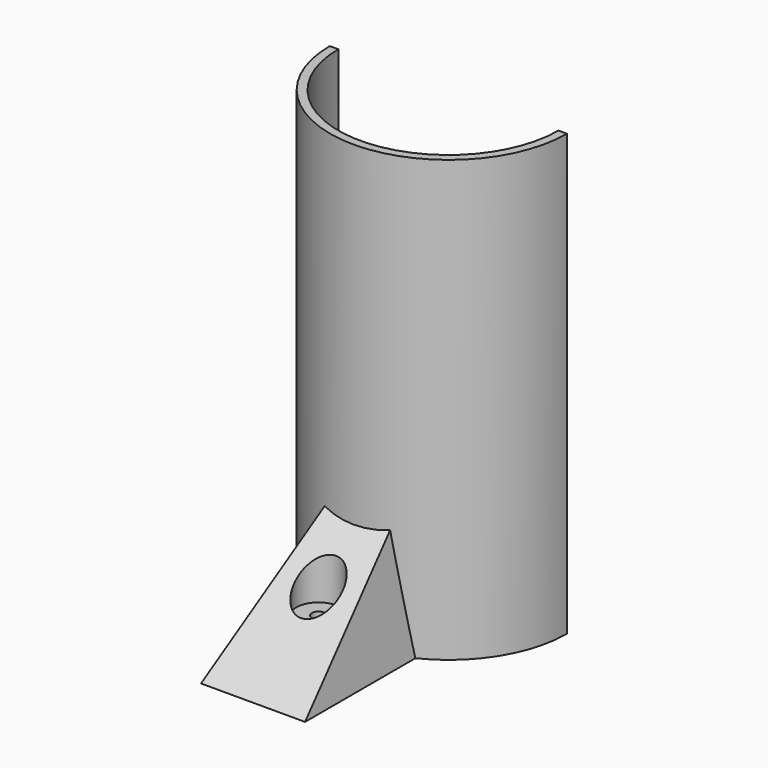
from build123d import *

# Parameters (mm, degrees)
F1_DEPTH               = 50
F2_DEPTH               = 50
DRAFT_F2_DRAFTED_ANGLE = -10
F3_T4_DEPTH            = 268.8954225412
F3_S5_R                = 26.9444420433
F3_T6_DEPTH            = 142
F4_D                   = 3
F4_DEPTH               = 50
F4_START               = 38.598583
F4_CBORE_D             = 10
F4_CBORE_DEPTH         = 1.5
F4_TIP                 = 0.9012909285
F5_D                   = 50
F5_DEPTH               = 50
F5_TIP                 = 15.0215154757


# Not quite as in the source:
# - a fillet or chamfer that OpenCascade refuses, or shapes differently, is made with other operations: its cross-section is extruded or revolved along the edge and cut away or added
# - an extrude with a draft is written as a straight extrude whose walls are then drafted
# - a feature names something its author has since deleted; it is built from what else it names


with BuildPart() as f1:
    # F0 (on Top) → F1 (new body, symmetric)
    with BuildSketch(Plane.XY):
        with BuildLine():
            Line((-25, 0), (-26.9505840936, 0))
            ThreePointArc((-26.9505840936, 0), (-20.0709771471, -17.9283263754), (-3, -26.7223935575))
            ThreePointArc((-3, -26.7223935575), (3.8782e-05, -26.8892302381), (3, -26.721004611))
            ThreePointArc((3, -26.721004611), (20.0627424058, -17.9236810762), (26.9381868614, 0))
            Line((26.9381868614, 0), (25, 0))
            ThreePointArc((25, 0), (0, -25), (-25, 0))
        make_face()
    extrude(amount=F1_DEPTH, both=True)


with BuildPart() as f2_drafted:
    # F0 (on Top) → F2 (new body)
    with BuildSketch(Plane.XY):
        with BuildLine():
            ThreePointArc((3, -26.721004611), (3.8782e-05, -26.8892302381), (-3, -26.7223935575))
            Line((-3, -26.7223935575), (-3, -46.88923096))
            Line((-3, -46.88923096), (0, -46.88923096))
            Line((0, -46.88923096), (3, -46.88923096))
            Line((3, -46.88923096), (3, -26.721004611))
        make_face()
    extrude(amount=-F2_DEPTH)

    # draft_F2_drafted
    draft_f2_drafted_walls = [f2_drafted.faces().sort_by_distance(p)[0] for p in [
        (3.8782e-05, -26.8892302381, -33.3333333333),
        (0, -46.88923096, -33.3333333333),
        (-3, -36.8058122588, -33.3333333333),
        (3, -36.8051177855, -33.3333333333),
    ]]
    draft(draft_f2_drafted_walls, neutral_plane=Plane(origin=(0, 0, 0), x_dir=(1, 0, 0), z_dir=(0, 0, -1)), angle=DRAFT_F2_DRAFTED_ANGLE)


with BuildPart() as f1_1:
    add(f1.part)

    # join_F2_drafted: union F2_drafted
    add(f2_drafted.part)

    # F3: chamfer of 51 on 1 edges, made by hand


with BuildPart() as f3_tool2:
    # F3_s3 → F3_t4 (new body)
    with BuildSketch(Plane.YZ.offset(134.4477112706)):
        with BuildLine():
            Line((5.6734997039, 1.3112867238), (-57.308018685, -51.5364821274))
            Line((-57.308018685, -51.5364821274), (-58.3125225931, -51.3593609862))
            ThreePointArc((-58.3125225931, -51.3593609862), (-52.4574460646, -25.7049711975), (-47.8937348681, 0.1771211412))
            Line((-47.8937348681, 0.1771211412), (-46.88923096, 1.02))
            ThreePointArc((-46.88923096, 1.02), (-20.6078656281, 1.02), (5.6734997039, 2.3312867238))
            Line((5.6734997039, 2.3312867238), (5.6734997039, 1.3112867238))
        make_face()
    extrude(amount=-F3_T4_DEPTH)

    # F3_s5 → F3_t6 (cut, symmetric)
    with BuildSketch(Plane.XY.offset(-24.6)):
        with Locations((-0.0061986161, 0.0552110832)):
            Circle(F3_S5_R)
    extrude(amount=F3_T6_DEPTH, both=True, mode=Mode.SUBTRACT)

    split(bisect_by=Plane(origin=(2.9095389312, 0, 0.513030215), x_dir=(0, 1, 0), z_dir=(-0.984807753, 0, -0.1736481777)), keep=Keep.TOP)

    split(bisect_by=Plane(origin=(-2.9095389312, 0, 0.513030215), x_dir=(0, 1, 0), z_dir=(0.984807753, 0, -0.1736481777)), keep=Keep.TOP)


with BuildPart() as f1_2:
    add(f1_1.part)

    # F3_t1: cut F3_tool2
    add(f3_tool2.part, mode=Mode.SUBTRACT)

    # F4
    # its depths count from where the whole tool has entered the part; down to there all is cleared
    with Locations(Plane.XY.offset(-F4_START)):
        with Locations((0, -36.88923096)):
            CounterBoreHole(F4_D / 2, F4_CBORE_D / 2, F4_CBORE_DEPTH, depth=F4_DEPTH)
            with Locations((0, 0, -(F4_DEPTH + F4_TIP / 2))):  # 118° drill point
                Cone(0, F4_D / 2, F4_TIP, mode=Mode.SUBTRACT)

    # F5
    with Locations(Plane.XY):
        with Locations((0, 0)):
            Hole(F5_D / 2, depth=F5_DEPTH)
            with Locations((0, 0, -(F5_DEPTH + F5_TIP / 2))):  # 118° drill point
                Cone(0, F5_D / 2, F5_TIP, mode=Mode.SUBTRACT)


solid = f1_2.part
